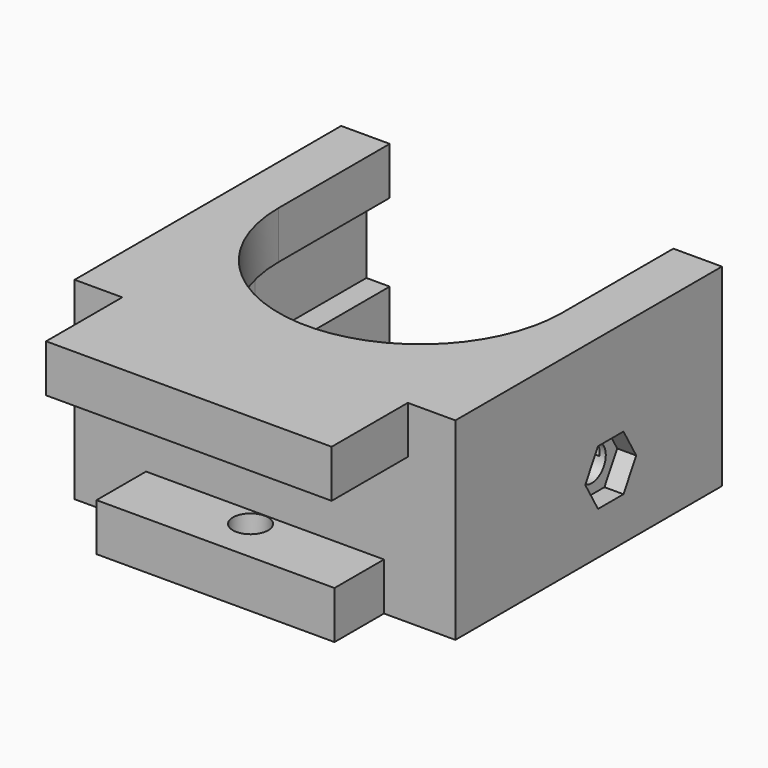
from build123d import *

# Parameters (mm, degrees)
F0_W      = 25
F0_H      = 6.5
F0_R      = 1.85
F1_DEPTH  = 5
F3_DEPTH  = 2.1
F5_DEPTH  = 8.2
F7_DEPTH  = 5
F9_DEPTH  = 2
F11_DEPTH = 2
F12_R     = 1.85
F13_DEPTH = 5
F14_R     = 1.85
F15_DEPTH = 5
F17_DEPTH = 2


# Not quite as in the source:
# - a feature names something its author has since deleted; it is built from what else it names


with BuildPart() as f1:
    # F0 (on Top) → F1 (new body)
    with BuildSketch(Plane.XY):
        with BuildLine():
            Line((-14.9, 24), (-20, 24))
            Line((-20, 24), (-20, -11))
            Line((-20, -11), (-12.5, -11))
            Line((-12.5, -11), (12.5, -11))
            Line((12.5, -11), (20, -11))
            Line((20, -11), (20, 24))
            Line((20, 24), (14.9, 24))
            Line((14.9, 24), (14.9, 9.4))
            ThreePointArc((14.9, 9.4), (0, -5.5), (-14.9, 9.4))
            Line((-14.9, 9.4), (-14.9, 24))
        make_face()
        with Locations((0, -14.25)):
            Rectangle(F0_W, F0_H)
        with Locations((0, -12.9)):
            Circle(F0_R, mode=Mode.SUBTRACT)
    extrude(amount=F1_DEPTH)

    # F2 (on face) → F3 (join)
    with BuildSketch(Plane.XY.offset(5)):
        with BuildLine():
            Line((-14.9, 24), (-20, 24))
            Line((-20, 24), (-20, -11))
            Line((-20, -11), (20, -11))
            Line((20, -11), (20, 24))
            Line((20, 24), (14.9, 24))
            Line((14.9, 24), (14.9, 9.4))
            ThreePointArc((14.9, 9.4), (0, -5.5), (-14.9, 9.4))
            Line((-14.9, 9.4), (-14.9, 24))
        make_face()
    extrude(amount=F3_DEPTH)

    # F4 (on face) → F5 (join)
    with BuildSketch(Plane.XY.offset(7.1)):
        with BuildLine():
            Line((-17.35, 24), (-20, 24))
            Line((-20, 24), (-20, -11))
            Line((-20, -11), (20, -11))
            Line((20, -11), (20, 24))
            Line((20, 24), (17.35, 24))
            Line((17.35, 24), (17.35, 9.4))
            ThreePointArc((17.35, 9.4), (0, -7.95), (-17.35, 9.4))
            Line((-17.35, 9.4), (-17.35, 24))
        make_face()
    extrude(amount=F5_DEPTH)

    # F6 (on face) → F7 (join)
    with BuildSketch(Plane.XY.offset(15.3)):
        with BuildLine():
            Line((-14.9, 24), (-20, 24))
            Line((-20, 24), (-20, -11))
            Line((-20, -11), (-15, -11))
            Line((-15, -11), (-15, -21))
            Line((-15, -21), (15, -21))
            Line((15, -21), (15, -11))
            Line((15, -11), (20, -11))
            Line((20, -11), (20, 24))
            Line((20, 24), (14.9, 24))
            Line((14.9, 24), (14.9, 9.4))
            ThreePointArc((14.9, 9.4), (0, -5.5), (-14.9, 9.4))
            Line((-14.9, 9.4), (-14.9, 24))
        make_face()
    extrude(amount=F7_DEPTH)

    # F8 (on face) → F9 (cut)
    with BuildSketch(Plane(origin=(-20, 0, 0), x_dir=(0, -1, 0), z_dir=(-1, 0, 0))):
        with BuildLine():
            ThreePointArc((-6.8885265259, 5.9499996589), (-6.5988151547, 6.649424579), (-6.5, 7.4))
            ThreePointArc((-6.5, 7.4), (-6.598815139, 8.1505753623), (-6.8885264651, 8.8500002357))
            ThreePointArc((-6.8885264651, 8.8500002357), (-7.9500001179, 9.911473739), (-9.4, 10.3))
            ThreePointArc((-9.4, 10.3), (-10.849999907, 9.9114737247), (-11.9114735636, 8.850000186))
            ThreePointArc((-11.9114735636, 8.850000186), (-12.3, 7.3999999856), (-11.9114735492, 5.9499997892))
            ThreePointArc((-11.9114735492, 5.9499997892), (-10.8499998946, 4.8885262682), (-9.4, 4.5))
            ThreePointArc((-9.4, 4.5), (-7.9500001705, 4.8885262306), (-6.8885265259, 5.9499996589))
        make_face()
        with BuildLine():
            ThreePointArc((-6.8885264651, 8.8500002357), (-6.598815139, 8.1505753623), (-6.5, 7.4))
            ThreePointArc((-6.5, 7.4), (-6.5988151547, 6.649424579), (-6.8885265259, 5.9499996589))
            Line((-6.8885265259, 5.9499996589), (-6.0513684387, 7.4))
            Line((-6.0513684387, 7.4), (-6.8885264651, 8.8500002357))
        make_face()
        with BuildLine():
            ThreePointArc((-9.4, 10.3), (-7.9500001179, 9.911473739), (-6.8885264651, 8.8500002357))
            Line((-6.8885264651, 8.8500002357), (-7.7256842194, 10.3))
            Line((-7.7256842194, 10.3), (-9.4, 10.3))
        make_face()
        with BuildLine():
            Line((-7.7256842194, 4.5), (-6.8885265259, 5.9499996589))
            ThreePointArc((-6.8885265259, 5.9499996589), (-7.9500001705, 4.8885262306), (-9.4, 4.5))
            Line((-9.4, 4.5), (-7.7256842194, 4.5))
        make_face()
        with BuildLine():
            ThreePointArc((-11.9114735636, 8.850000186), (-10.849999907, 9.9114737247), (-9.4, 10.3))
            Line((-9.4, 10.3), (-11.0743157806, 10.3))
            Line((-11.0743157806, 10.3), (-11.9114735636, 8.850000186))
        make_face()
        with BuildLine():
            Line((-11.0743157806, 4.5), (-9.4, 4.5))
            ThreePointArc((-9.4, 4.5), (-10.8499998946, 4.8885262682), (-11.9114735492, 5.9499997892))
            Line((-11.9114735492, 5.9499997892), (-11.0743157806, 4.5))
        make_face()
        with BuildLine():
            ThreePointArc((-11.9114735492, 5.9499997892), (-12.3, 7.3999999856), (-11.9114735636, 8.850000186))
            Line((-11.9114735636, 8.850000186), (-12.7486315613, 7.4))
            Line((-12.7486315613, 7.4), (-11.9114735492, 5.9499997892))
        make_face()
    extrude(amount=-F9_DEPTH, mode=Mode.SUBTRACT)

    # F10 (on face) → F11 (cut)
    with BuildSketch(Plane.YZ.offset(20)):
        Polygon((11.0743157806, 10.3), (7.7256842194, 10.3), (6.0513684387, 7.4), (7.7256842194, 4.5), (11.0743157806, 4.5), (12.7486315613, 7.4), align=None)
    extrude(amount=-F11_DEPTH, mode=Mode.SUBTRACT)

    # F12 (on face) → F13 (cut)
    with BuildSketch(Plane.YZ.offset(18)):
        with Locations((9.4, 7.4)):
            Circle(F12_R)
    extrude(amount=-F13_DEPTH, mode=Mode.SUBTRACT)

    # F14 (on face) → F15 (cut)
    with BuildSketch(Plane(origin=(-18, 0, 0), x_dir=(0, -1, 0), z_dir=(-1, 0, 0))):
        with Locations((-9.4, 7.4)):
            Circle(F14_R)
    extrude(amount=-F15_DEPTH, mode=Mode.SUBTRACT)

    # F16 (on Top) → F17 (cut)
    with BuildSketch(Plane.XY):
        Polygon((-1.6743157806, -15.8), (1.6743157806, -15.8), (3.3486315613, -12.9), (1.6743157806, -10), (-1.6743157806, -10), (-3.3486315613, -12.9), align=None)
    extrude(amount=F17_DEPTH, mode=Mode.SUBTRACT)


solid = f1.part
